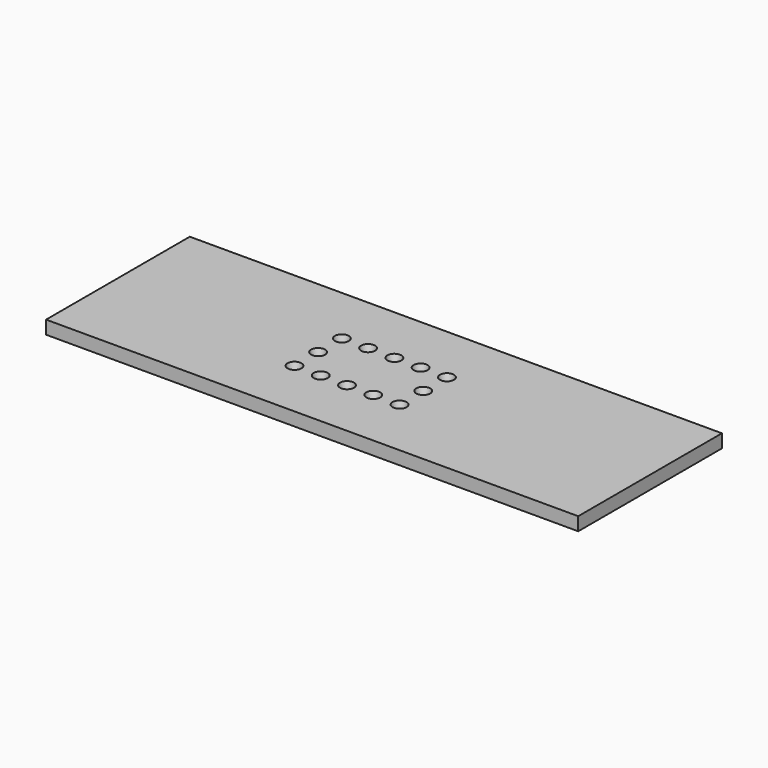
from build123d import *

# Parameters (mm, degrees)
F0_W                      = 80
F0_H                      = 27
F1_DEPTH                  = 2
F2_R                      = 1.05
F3_DEPTH                  = 25
DRAFT_F3_DRAFTED_ANGLE    = 14
DRAFT_F3_2_DRAFTED_ANGLE  = 14
DRAFT_F3_3_DRAFTED_ANGLE  = 14
DRAFT_F3_4_DRAFTED_ANGLE  = 14
DRAFT_F3_5_DRAFTED_ANGLE  = 14
DRAFT_F3_6_DRAFTED_ANGLE  = 14
DRAFT_F3_7_DRAFTED_ANGLE  = 14
DRAFT_F3_8_DRAFTED_ANGLE  = 14
DRAFT_F3_9_DRAFTED_ANGLE  = 14
DRAFT_F3_10_DRAFTED_ANGLE = 14
DRAFT_F3_11_DRAFTED_ANGLE = 14
DRAFT_F3_12_DRAFTED_ANGLE = 14


# Not quite as in the source:
# - an extrude with a draft is written as a straight extrude whose walls are then drafted


with BuildPart() as f1:
    # F0 (on Top) → F1 (new body)
    with BuildSketch(Plane.XY):
        Rectangle(F0_W, F0_H)
    extrude(amount=F1_DEPTH)


with BuildPart() as f3_drafted:
    # F2 (on face) → F3 (new body)
    with BuildSketch(Plane.XY.offset(2)):
        with Locations((-9.9, 4.45)):
            Circle(F2_R)
    extrude(amount=-F3_DEPTH)

    # draft_F3_drafted
    draft_f3_drafted_walls = [f3_drafted.faces().sort_by_distance(p)[0] for p in [
        (-10.95, 4.45, -14.6666666667),
    ]]
    draft(draft_f3_drafted_walls, neutral_plane=Plane(origin=(0, 0, 2), x_dir=(1, 0, 0), z_dir=(0, 0, -1)), angle=DRAFT_F3_DRAFTED_ANGLE)


with BuildPart() as f1_1:
    add(f1.part)

    # join_F3_drafted: cut F3_drafted
    add(f3_drafted.part, mode=Mode.SUBTRACT)


with BuildPart() as f3_2_drafted:
    # F2 (on face) → F3, piece 2 (new body)
    with BuildSketch(Plane.XY.offset(2)):
        with Locations((-5.95, 4.45)):
            Circle(F2_R)
    extrude(amount=-F3_DEPTH)

    # draft_F3_2_drafted
    draft_f3_2_drafted_walls = [f3_2_drafted.faces().sort_by_distance(p)[0] for p in [
        (-7, 4.45, -14.6666666667),
    ]]
    draft(draft_f3_2_drafted_walls, neutral_plane=Plane(origin=(0, 0, 2), x_dir=(1, 0, 0), z_dir=(0, 0, -1)), angle=DRAFT_F3_2_DRAFTED_ANGLE)


with BuildPart() as f1_2:
    add(f1_1.part)

    # join_F3_2_drafted: cut F3_2_drafted
    add(f3_2_drafted.part, mode=Mode.SUBTRACT)


with BuildPart() as f3_3_drafted:
    # F2 (on face) → F3, piece 3 (new body)
    with BuildSketch(Plane.XY.offset(2)):
        with Locations((-2, 4.45)):
            Circle(F2_R)
    extrude(amount=-F3_DEPTH)

    # draft_F3_3_drafted
    draft_f3_3_drafted_walls = [f3_3_drafted.faces().sort_by_distance(p)[0] for p in [
        (-3.05, 4.45, -14.6666666667),
    ]]
    draft(draft_f3_3_drafted_walls, neutral_plane=Plane(origin=(0, 0, 2), x_dir=(1, 0, 0), z_dir=(0, 0, -1)), angle=DRAFT_F3_3_DRAFTED_ANGLE)


with BuildPart() as f1_3:
    add(f1_2.part)

    # join_F3_3_drafted: cut F3_3_drafted
    add(f3_3_drafted.part, mode=Mode.SUBTRACT)


with BuildPart() as f3_4_drafted:
    # F2 (on face) → F3, piece 4 (new body)
    with BuildSketch(Plane.XY.offset(2)):
        with Locations((1.95, 4.45)):
            Circle(F2_R)
    extrude(amount=-F3_DEPTH)

    # draft_F3_4_drafted
    draft_f3_4_drafted_walls = [f3_4_drafted.faces().sort_by_distance(p)[0] for p in [
        (0.9, 4.45, -14.6666666667),
    ]]
    draft(draft_f3_4_drafted_walls, neutral_plane=Plane(origin=(0, 0, 2), x_dir=(1, 0, 0), z_dir=(0, 0, -1)), angle=DRAFT_F3_4_DRAFTED_ANGLE)


with BuildPart() as f1_4:
    add(f1_3.part)

    # join_F3_4_drafted: cut F3_4_drafted
    add(f3_4_drafted.part, mode=Mode.SUBTRACT)


with BuildPart() as f3_5_drafted:
    # F2 (on face) → F3, piece 5 (new body)
    with BuildSketch(Plane.XY.offset(2)):
        with Locations((5.9, 4.45)):
            Circle(F2_R)
    extrude(amount=-F3_DEPTH)

    # draft_F3_5_drafted
    draft_f3_5_drafted_walls = [f3_5_drafted.faces().sort_by_distance(p)[0] for p in [
        (4.85, 4.45, -14.6666666667),
    ]]
    draft(draft_f3_5_drafted_walls, neutral_plane=Plane(origin=(0, 0, 2), x_dir=(1, 0, 0), z_dir=(0, 0, -1)), angle=DRAFT_F3_5_DRAFTED_ANGLE)


with BuildPart() as f1_5:
    add(f1_4.part)

    # join_F3_5_drafted: cut F3_5_drafted
    add(f3_5_drafted.part, mode=Mode.SUBTRACT)


with BuildPart() as f3_6_drafted:
    # F2 (on face) → F3, piece 6 (new body)
    with BuildSketch(Plane.XY.offset(2)):
        with Locations((-9.9, 0)):
            Circle(F2_R)
    extrude(amount=-F3_DEPTH)

    # draft_F3_6_drafted
    draft_f3_6_drafted_walls = [f3_6_drafted.faces().sort_by_distance(p)[0] for p in [
        (-10.95, 0, -14.6666666667),
    ]]
    draft(draft_f3_6_drafted_walls, neutral_plane=Plane(origin=(0, 0, 2), x_dir=(1, 0, 0), z_dir=(0, 0, -1)), angle=DRAFT_F3_6_DRAFTED_ANGLE)


with BuildPart() as f1_6:
    add(f1_5.part)

    # join_F3_6_drafted: cut F3_6_drafted
    add(f3_6_drafted.part, mode=Mode.SUBTRACT)


with BuildPart() as f3_7_drafted:
    # F2 (on face) → F3, piece 7 (new body)
    with BuildSketch(Plane.XY.offset(2)):
        with Locations((-5.95, -4.45)):
            Circle(F2_R)
    extrude(amount=-F3_DEPTH)

    # draft_F3_7_drafted
    draft_f3_7_drafted_walls = [f3_7_drafted.faces().sort_by_distance(p)[0] for p in [
        (-7, -4.45, -14.6666666667),
    ]]
    draft(draft_f3_7_drafted_walls, neutral_plane=Plane(origin=(0, 0, 2), x_dir=(1, 0, 0), z_dir=(0, 0, -1)), angle=DRAFT_F3_7_DRAFTED_ANGLE)


with BuildPart() as f1_7:
    add(f1_6.part)

    # join_F3_7_drafted: cut F3_7_drafted
    add(f3_7_drafted.part, mode=Mode.SUBTRACT)


with BuildPart() as f3_8_drafted:
    # F2 (on face) → F3, piece 8 (new body)
    with BuildSketch(Plane.XY.offset(2)):
        with Locations((-2, -4.45)):
            Circle(F2_R)
    extrude(amount=-F3_DEPTH)

    # draft_F3_8_drafted
    draft_f3_8_drafted_walls = [f3_8_drafted.faces().sort_by_distance(p)[0] for p in [
        (-3.05, -4.45, -14.6666666667),
    ]]
    draft(draft_f3_8_drafted_walls, neutral_plane=Plane(origin=(0, 0, 2), x_dir=(1, 0, 0), z_dir=(0, 0, -1)), angle=DRAFT_F3_8_DRAFTED_ANGLE)


with BuildPart() as f1_8:
    add(f1_7.part)

    # join_F3_8_drafted: cut F3_8_drafted
    add(f3_8_drafted.part, mode=Mode.SUBTRACT)


with BuildPart() as f3_9_drafted:
    # F2 (on face) → F3, piece 9 (new body)
    with BuildSketch(Plane.XY.offset(2)):
        with Locations((-9.9, -4.45)):
            Circle(F2_R)
    extrude(amount=-F3_DEPTH)

    # draft_F3_9_drafted
    draft_f3_9_drafted_walls = [f3_9_drafted.faces().sort_by_distance(p)[0] for p in [
        (-10.95, -4.45, -14.6666666667),
    ]]
    draft(draft_f3_9_drafted_walls, neutral_plane=Plane(origin=(0, 0, 2), x_dir=(1, 0, 0), z_dir=(0, 0, -1)), angle=DRAFT_F3_9_DRAFTED_ANGLE)


with BuildPart() as f1_9:
    add(f1_8.part)

    # join_F3_9_drafted: cut F3_9_drafted
    add(f3_9_drafted.part, mode=Mode.SUBTRACT)


with BuildPart() as f3_10_drafted:
    # F2 (on face) → F3, piece 10 (new body)
    with BuildSketch(Plane.XY.offset(2)):
        with Locations((1.95, -4.45)):
            Circle(F2_R)
    extrude(amount=-F3_DEPTH)

    # draft_F3_10_drafted
    draft_f3_10_drafted_walls = [f3_10_drafted.faces().sort_by_distance(p)[0] for p in [
        (0.9, -4.45, -14.6666666667),
    ]]
    draft(draft_f3_10_drafted_walls, neutral_plane=Plane(origin=(0, 0, 2), x_dir=(1, 0, 0), z_dir=(0, 0, -1)), angle=DRAFT_F3_10_DRAFTED_ANGLE)


with BuildPart() as f1_10:
    add(f1_9.part)

    # join_F3_10_drafted: cut F3_10_drafted
    add(f3_10_drafted.part, mode=Mode.SUBTRACT)


with BuildPart() as f3_11_drafted:
    # F2 (on face) → F3, piece 11 (new body)
    with BuildSketch(Plane.XY.offset(2)):
        with Locations((5.9, -4.45)):
            Circle(F2_R)
    extrude(amount=-F3_DEPTH)

    # draft_F3_11_drafted
    draft_f3_11_drafted_walls = [f3_11_drafted.faces().sort_by_distance(p)[0] for p in [
        (4.85, -4.45, -14.6666666667),
    ]]
    draft(draft_f3_11_drafted_walls, neutral_plane=Plane(origin=(0, 0, 2), x_dir=(1, 0, 0), z_dir=(0, 0, -1)), angle=DRAFT_F3_11_DRAFTED_ANGLE)


with BuildPart() as f1_11:
    add(f1_10.part)

    # join_F3_11_drafted: cut F3_11_drafted
    add(f3_11_drafted.part, mode=Mode.SUBTRACT)


with BuildPart() as f3_12_drafted:
    # F2 (on face) → F3, piece 12 (new body)
    with BuildSketch(Plane.XY.offset(2)):
        with Locations((5.9, 0)):
            Circle(F2_R)
    extrude(amount=-F3_DEPTH)

    # draft_F3_12_drafted
    draft_f3_12_drafted_walls = [f3_12_drafted.faces().sort_by_distance(p)[0] for p in [
        (4.85, 0, -14.6666666667),
    ]]
    draft(draft_f3_12_drafted_walls, neutral_plane=Plane(origin=(0, 0, 2), x_dir=(1, 0, 0), z_dir=(0, 0, -1)), angle=DRAFT_F3_12_DRAFTED_ANGLE)


with BuildPart() as f1_12:
    add(f1_11.part)

    # join_F3_12_drafted: cut F3_12_drafted
    add(f3_12_drafted.part, mode=Mode.SUBTRACT)


solid = f1_12.part
